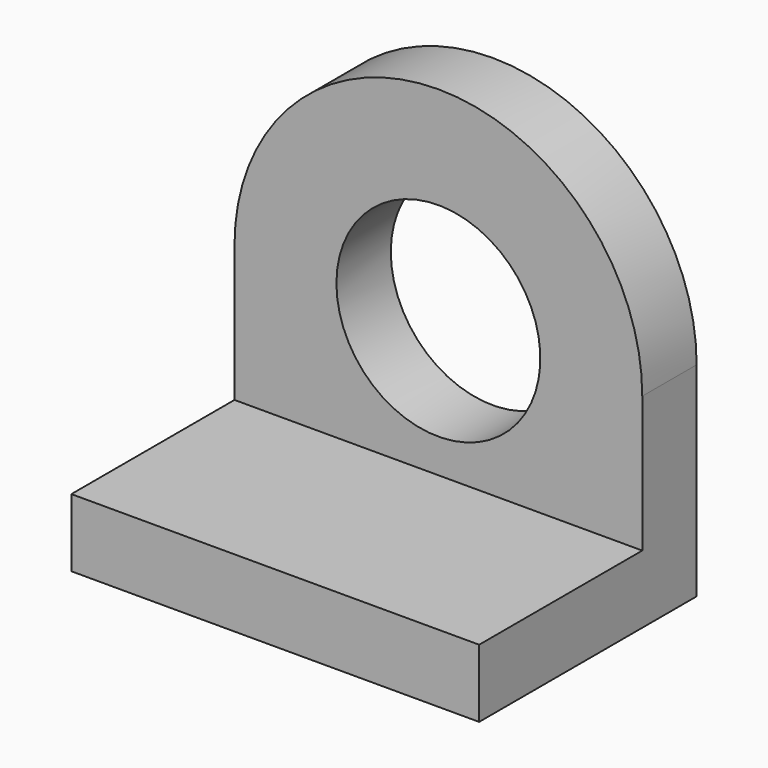
from build123d import *

# Parameters (mm, degrees)
F0_W     = 76.2
F0_H     = 50.8
F1_DEPTH = 12.7
F2_W     = 12.7
F2_H     = 25.4
F3_DEPTH = 76.2
F5_DEPTH = 12.7
F7_DEPTH = 30.48


with BuildPart() as f1:
    # F0 (on Top) → F1 (new body)
    with BuildSketch(Plane.XY):
        with Locations((-38.1, 25.4)):
            Rectangle(F0_W, F0_H)
    extrude(amount=F1_DEPTH)

    # F2 (on face) → F3 (join)
    with BuildSketch(Plane.YZ):
        with Locations((44.45, 25.4)):
            Rectangle(F2_W, F2_H)
    extrude(amount=-F3_DEPTH)

    # F4 (on face) → F5 (join)
    with BuildSketch(Plane.XZ.offset(-38.1)):
        with BuildLine():
            Line((-19.05, 38.1), (0, 38.1))
            ThreePointArc((0, 38.1), (-38.1, 76.2), (-76.2, 38.1))
            Line((-76.2, 38.1), (-57.15, 38.1))
            ThreePointArc((-57.15, 38.1), (-38.1, 57.15), (-19.05, 38.1))
        make_face()
    extrude(amount=-F5_DEPTH)

    # F6 (on face) → F7 (cut)
    with BuildSketch(Plane.XZ.offset(-38.1)):
        with BuildLine():
            Line((-57.15, 38.1), (-19.05, 38.1))
            ThreePointArc((-19.05, 38.1), (-38.1, 57.15), (-57.15, 38.1))
        make_face()
        with BuildLine():
            ThreePointArc((-57.15, 38.1), (-38.1, 19.05), (-19.05, 38.1))
            Line((-19.05, 38.1), (-57.15, 38.1))
        make_face()
    extrude(amount=-F7_DEPTH, mode=Mode.SUBTRACT)


solid = f1.part
